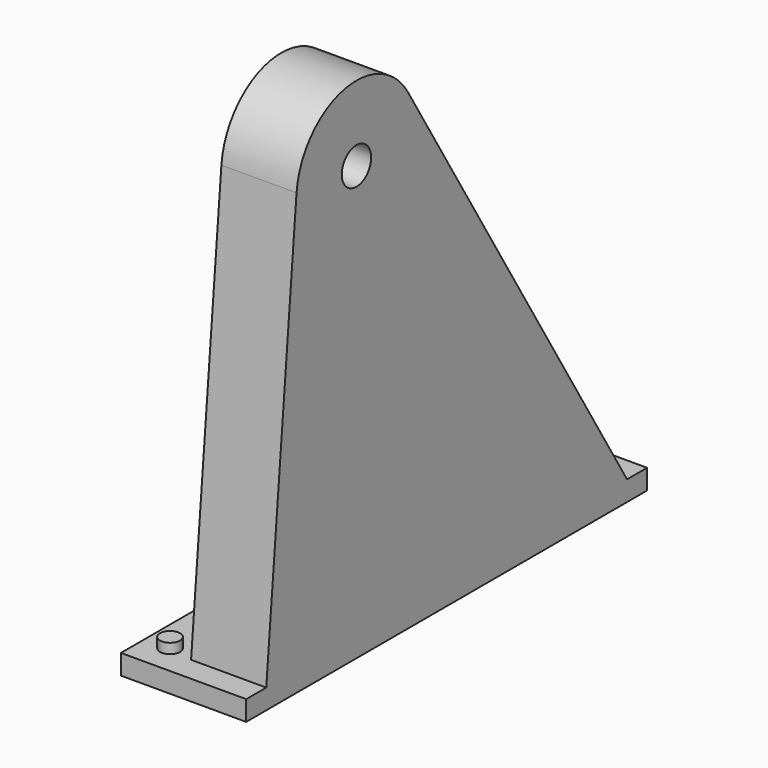
from build123d import *

# Parameters (mm, degrees)
F1_W          = 30
F1_H          = 1.2
F2_DEPTH      = 4.5
F2_DEPTH_BACK = 3
F3_R          = 1.1
F4_DEPTH      = 4.5
F6_DEPTH      = 2.25
F7_R          = 3
F8_R          = 2.24999
F9_R          = 0.6
F10_DEPTH     = 0.6


# Not quite as in the source:
# - a fillet or chamfer is up to 0.001 mm smaller than in the source, because OpenCascade refuses the exact size


with BuildPart() as f2:
    # F1 (on Right) → F2 (new body, two sides)
    with BuildSketch(Plane.YZ) as f2_sk:
        with Locations((6.75, 0.6)):
            Rectangle(F1_W, F1_H)
    extrude(amount=F2_DEPTH)
    extrude(f2_sk.sketch, amount=-F2_DEPTH_BACK)

    # F3 (on Right) → F4 (join)
    with BuildSketch(Plane.YZ):
        with BuildLine():
            Line((-6.75, 1.2), (20.25, 1.2))
            Line((20.25, 1.2), (3.8491422789, 28.28111641))
            ThreePointArc((3.8491422789, 28.28111641), (-1.0140939829, 30.3342460462), (-4.4818163226, 26.3541317243))
            Line((-4.4818163226, 26.3541317243), (-6.75, 1.2))
        make_face()
        with Locations((0, 25.95)):
            Circle(F3_R, mode=Mode.SUBTRACT)
    extrude(amount=F4_DEPTH)

    # F5 (on face) → F6 (cut)
    with BuildSketch(Plane(origin=(0, 0, 0), x_dir=(0, -1, 0), z_dir=(-1, 0, 0))):
        Polygon((-13.8610392149, 4.8), (2.8107769402, 4.8), (1.3229485752, 21.3), (-3.8683140886, 21.3), align=None)
    extrude(amount=-F6_DEPTH, mode=Mode.SUBTRACT)

    # F7
    f7_edges = [f2.edges().sort_by_distance(p)[0] for p in [
        (1.125, -1.322949, 21.3),
        (1.125, 3.868314, 21.3),
        (1.125, 13.861039, 4.8),
        (1.125, -2.810777, 4.8),
    ]]
    fillet(f7_edges, radius=F7_R)

    # F8 (radius 2.25 in the source; OpenCascade refuses exactly that, so slightly less here)
    f8_edges = [f2.edges().sort_by_distance(p)[0] for p in [
        (2.25, 4.504407, 4.8),
        (2.25, 11.150546, 6.327287),
        (2.25, -1.742618, 5.776175),
        (2.25, 7.923497, 14.604078),
        (2.25, -2.042569, 13.319421),
        (2.25, 3.650611, 20.91364),
        (2.25, -0.605116, 20.514527),
        (2.25, 1.798304, 21.3),
    ]]
    fillet(f8_edges, radius=F8_R)

    # F9 (on face) → F10 (join)
    with BuildSketch(Plane.XY.offset(1.2)):
        with Locations((-1.5, -6.45)):
            Circle(F9_R)
        with Locations((-1.5, -1.2)):
            Circle(F9_R)
        with Locations((-1.5, 4.05)):
            Circle(F9_R)
        with Locations((-1.5, 9.3)):
            Circle(F9_R)
        with Locations((-1.5, 14.55)):
            Circle(F9_R)
        with Locations((-1.5, 19.8)):
            Circle(F9_R)
    extrude(amount=F10_DEPTH)


solid = f2.part
